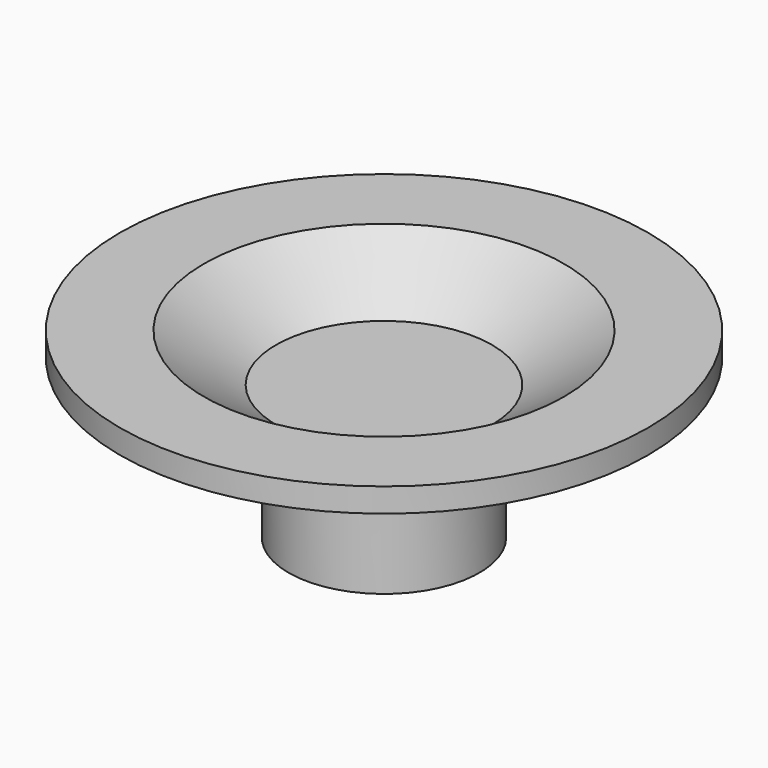
from build123d import *

# Parameters (mm, degrees)
F2_R     = 7.5
F3_DEPTH = 2
F4_SIZE2 = 1.99999
F4_SIZE  = 2.99999


# Not quite as in the source:
# - a fillet or chamfer is up to 0.001 mm smaller than in the source, because OpenCascade refuses the exact size


with BuildPart() as f1:
    # F0 (on Front) → F1 (revolve)
    with BuildSketch(Plane.XZ):
        Polygon((-3.975, 0), (0, 0), (0, 7.6), (-11, 7.6), (-11, 6.6), (-3.975, 3), align=None)
    revolve(axis=Axis((0, 0, 3.8), (0, 0, 1)))

    # F2 (on face) → F3 (cut)
    with BuildSketch(Plane.XY.offset(7.6)):
        Circle(F2_R)
    extrude(amount=-F3_DEPTH, mode=Mode.SUBTRACT)

    # F4 (size 3 and 2 in the source; OpenCascade refuses exactly that, so slightly less here)
    f4_edges = [f1.edges().sort_by_distance(p)[0] for p in [
        (-7.5, 0, 5.6),
    ]]
    f4_side = f1.faces().sort_by_distance((0, 0, 5.6))[0]
    chamfer(f4_edges, length=F4_SIZE, length2=F4_SIZE2, reference=f4_side)


solid = f1.part
